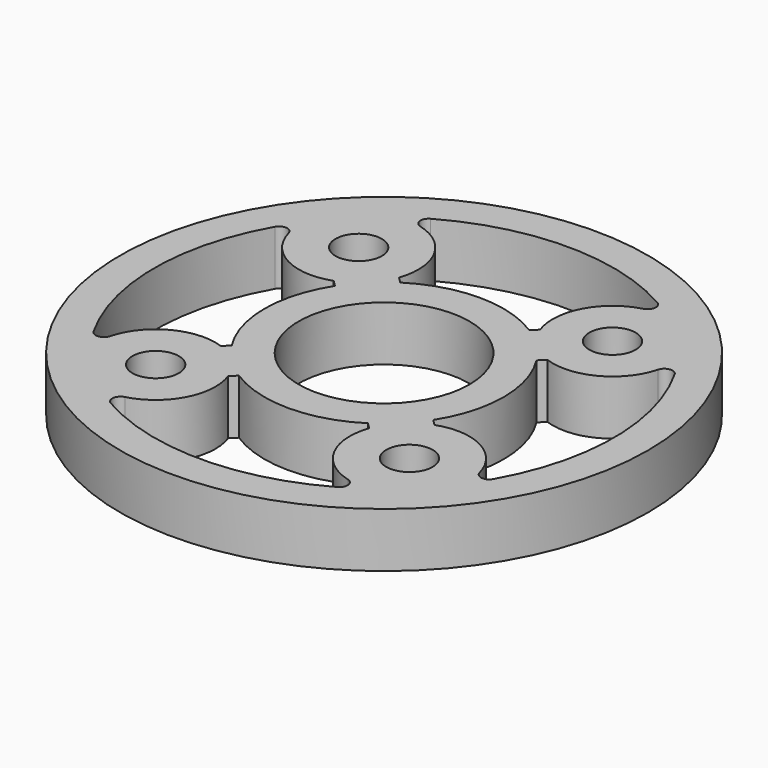
from build123d import *

# Parameters (mm, degrees)
F0_R            = 24.51608
F0_R_2          = 2.15265
F0_R_3          = 7.9375
F1_DEPTH        = 5.08
F3_DEPTH        = 5.08
F3_COPIES_COUNT = 4
F4_R            = 0.762


# Not quite as in the source:
# - a pattern or mirror of a feature is missing from the dataset's text; its kind, count and spacing are read off the source's solid


with BuildPart() as f1:
    # F0 (on Top) → F1 (new body)
    with BuildSketch(Plane.XY):
        Circle(F0_R)
        with Locations((-11.7865906, -11.7865906)):
            Circle(F0_R_2, mode=Mode.SUBTRACT)
        with Locations((11.7865906, -11.7865906)):
            Circle(F0_R_2, mode=Mode.SUBTRACT)
        with Locations((-11.7865906, 11.7865906)):
            Circle(F0_R_2, mode=Mode.SUBTRACT)
        Circle(F0_R_3, mode=Mode.SUBTRACT)
        with Locations((11.7865906, 11.7865906)):
            Circle(F0_R_2, mode=Mode.SUBTRACT)
    extrude(amount=F1_DEPTH)

    # F2 (on face) → F3 (cut, through all)
    with BuildSketch(Plane.XY.offset(5.08)):
        with BuildLine():
            ThreePointArc((-12.5005198818, 17.2967828873), (-7.4612395718, 15.2741760893), (-6.553034663, 9.9206307084))
            Line((-6.553034663, 9.9206307084), (-5.9913991959, 9.3589952413))
            ThreePointArc((-5.9913991959, 9.3589952413), (0, 11.1125), (5.9913991959, 9.3589952413))
            Line((5.9913991959, 9.3589952413), (6.553034663, 9.9206307084))
            ThreePointArc((6.553034663, 9.9206307084), (7.4612395718, 15.2741760893), (12.5005198818, 17.2967828873))
            ThreePointArc((12.5005198818, 17.2967828873), (0, 21.34108), (-12.5005198818, 17.2967828873))
        make_face()
    f3 = extrude(amount=-F3_DEPTH, mode=Mode.SUBTRACT)

    # F3_copies: F3 ×4 about axis
    f3_copies_axis = Axis((0, 0, 0), (0, 0, 1))
    for i in range(1, F3_COPIES_COUNT):
        add(f3.rotate(f3_copies_axis, i * 360 / F3_COPIES_COUNT), mode=Mode.SUBTRACT)

    # F4
    f4_edges = [f1.edges().sort_by_distance(p)[0] for p in [
        (-12.50052, 17.296783, 2.54),
        (12.50052, 17.296783, 2.54),
        (-17.296783, -12.50052, 2.54),
        (-17.296783, 12.50052, 2.54),
        (12.50052, -17.296783, 2.54),
        (-12.50052, -17.296783, 2.54),
        (17.296783, 12.50052, 2.54),
        (17.296783, -12.50052, 2.54),
    ]]
    fillet(f4_edges, radius=F4_R)


solid = f1.part
